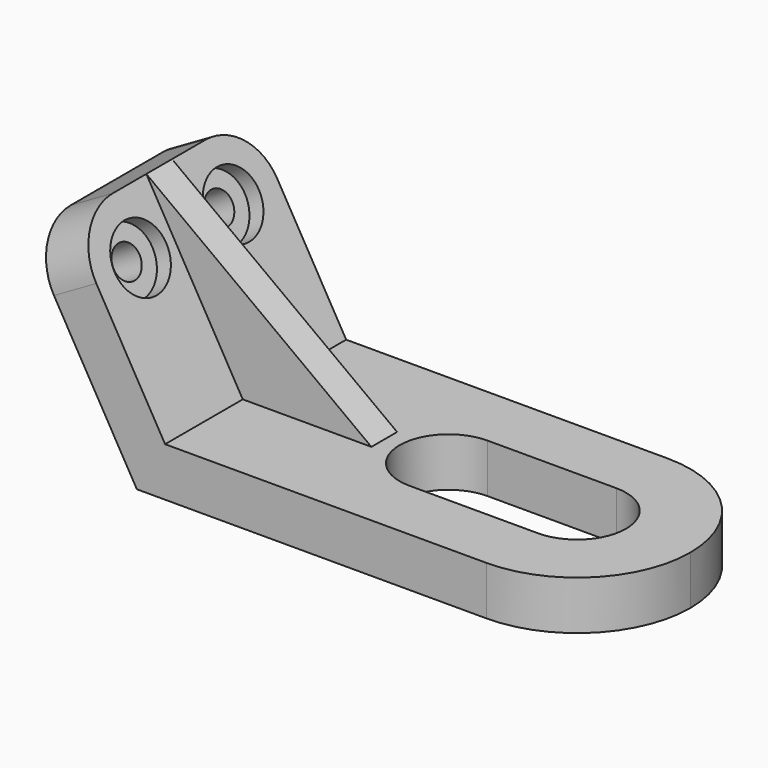
from build123d import *

# Parameters (mm, degrees)
F1_DEPTH      = 22.352
F1_DEPTH_BACK = 22.352
F3_DEPTH      = 3.175
F3_DEPTH_BACK = 3.175
F4_R          = 10.922
F5_R          = 22.35199
F7_DEPTH      = 9.652
F9_R          = 6.35
F9_R_2        = 3.175
F10_DEPTH     = 3.175
F11_DEPTH     = 28.5637839421
F12_R         = 6.35
F12_R_2       = 3.175
F13_DEPTH     = 3.1877
F14_DEPTH     = 28.5637839421


# Not quite as in the source:
# - a fillet or chamfer is up to 0.001 mm smaller than in the source, because OpenCascade refuses the exact size


with BuildPart() as f1:
    # F0 (on Front) → F1 (new body, two sides)
    with BuildSketch(Plane.XZ) as f1_sk:
        Polygon((-21.8362923991, 37.8215678842), (0, 0), (91.4245847982, 0), (91.4245847982, 9.652), (5.5725847982, 9.652), (-13.4774152018, 42.6475678842), align=None)
    extrude(amount=F1_DEPTH)
    extrude(f1_sk.sketch, amount=-F1_DEPTH_BACK)

    # F2 (on Front) → F3 (join, two sides)
    with BuildSketch(Plane.XZ) as f3_sk:
        Polygon((30.9725847982, 9.652), (-13.4774152018, 42.6475678842), (5.5725847982, 9.652), align=None)
    extrude(amount=F3_DEPTH)
    extrude(f3_sk.sketch, amount=-F3_DEPTH_BACK)

    # F4
    f4_edges = [f1.edges().sort_by_distance(p)[0] for p in [
        (-17.656854, -22.352, 40.234568),
        (-17.656854, 22.352, 40.234568),
    ]]
    fillet(f4_edges, radius=F4_R)

    # F5 (radius 22.352 in the source; OpenCascade refuses exactly that, so slightly less here)
    f5_edges = [f1.edges().sort_by_distance(p)[0] for p in [
        (91.424585, -22.352, 4.826),
        (91.424585, 22.352, 4.826),
    ]]
    fillet(f5_edges, radius=F5_R)

    # F6 (on face) → F7 (cut, through all)
    with BuildSketch(Plane.XY.offset(9.652)):
        with BuildLine():
            Line((43.6725847982, -9.652), (69.0725847982, -9.652))
            ThreePointArc((69.0725847982, -9.652), (78.7245847982, 0), (69.0725847982, 9.652))
            Line((69.0725847982, 9.652), (43.6725847982, 9.652))
            ThreePointArc((43.6725847982, 9.652), (34.0205847982, 0), (43.6725847982, -9.652))
        make_face()
    extrude(amount=-F7_DEPTH, mode=Mode.SUBTRACT)

    # F9 (on face) → F10 (cut)
    with BuildSketch(Plane(origin=(8.3588771973, 0, 4.826), x_dir=(0, 1, 0), z_dir=(0.8660254038, 0, 0.5))):
        with Locations((-11.43, 32.7505847982)):
            Circle(F9_R)
        with Locations((-11.43, 32.7505847982)):
            Circle(F9_R_2, mode=Mode.SUBTRACT)
        with Locations((-11.43, 32.7505847982)):
            Circle(F9_R_2)
    extrude(amount=-F10_DEPTH, mode=Mode.SUBTRACT)

    # F9 (on face) → F11 (cut, through all)
    with BuildSketch(Plane(origin=(8.3588771973, 0, 4.826), x_dir=(0, 1, 0), z_dir=(0.8660254038, 0, 0.5))):
        with Locations((-11.43, 32.7505847982)):
            Circle(F9_R_2)
    extrude(amount=-F11_DEPTH, mode=Mode.SUBTRACT)

    # F12 (on face) → F13 (cut)
    with BuildSketch(Plane(origin=(8.3588771973, 0, 4.826), x_dir=(0, 1, 0), z_dir=(0.8660254038, 0, 0.5))):
        with Locations((11.43, 32.7505847982)):
            Circle(F12_R)
        with Locations((11.43, 32.7505847982)):
            Circle(F12_R_2, mode=Mode.SUBTRACT)
        with Locations((11.43, 32.7505847982)):
            Circle(F12_R_2)
    extrude(amount=-F13_DEPTH, mode=Mode.SUBTRACT)

    # F12 (on face) → F14 (cut, through all)
    with BuildSketch(Plane(origin=(8.3588771973, 0, 4.826), x_dir=(0, 1, 0), z_dir=(0.8660254038, 0, 0.5))):
        with Locations((11.43, 32.7505847982)):
            Circle(F12_R_2)
    extrude(amount=-F14_DEPTH, mode=Mode.SUBTRACT)


solid = f1.part
